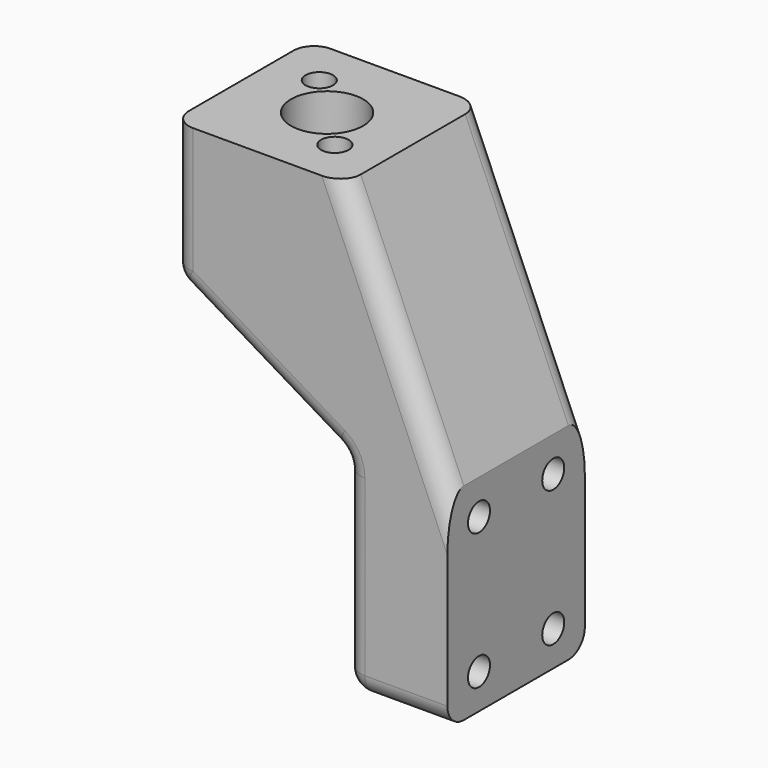
from build123d import *

# Parameters (mm, degrees)
F0_W      = 25
F0_H      = 20
F0_W_2    = 15
F0_H_2    = 30
F1_DEPTH  = 25
F2_R      = 5.25
F3_DEPTH  = 65.001
F4_R      = 2
F5_DEPTH  = 25
F6_R      = 3
F7_R      = 2
F8_DEPTH  = 65.001
F9_R      = 3.25
F10_DEPTH = 55.001


with BuildPart() as f1:
    # F0 (on Front) → F1 (new body)
    with BuildSketch(Plane.XZ):
        Polygon((12.5, 10), (12.5, -10), (-12.5, -10), (12.5, -25), (27.5, -25), align=None)
        Rectangle(F0_W, F0_H)
        with Locations((20, -40)):
            Rectangle(F0_W_2, F0_H_2)
    extrude(amount=F1_DEPTH)

    # F2 (on face) → F3 (cut, through all)
    with BuildSketch(Plane.XY.offset(10)):
        with Locations((0, -12.5)):
            Circle(F2_R)
    extrude(amount=-F3_DEPTH, mode=Mode.SUBTRACT)

    # F4 (on face) → F5 (cut)
    with BuildSketch(Plane(origin=(12.5, 0, 0), x_dir=(0, -1, 0), z_dir=(-1, 0, 0))):
        with Locations((19.25, -30.1)):
            Circle(F4_R)
        with Locations((5.75, -49.9)):
            Circle(F4_R)
        with Locations((5.75, -30.1)):
            Circle(F4_R)
        with Locations((19.25, -49.9)):
            Circle(F4_R)
    extrude(amount=-F5_DEPTH, mode=Mode.SUBTRACT)

    # F6
    f6_edges = [f1.edges().sort_by_distance(p)[0] for p in [
        (-12.5, -25, 0),
        (-12.5, 0, 0),
        (-12.5, -12.5, -10),
        (0, -25, -17.5),
        (0, 0, -17.5),
        (12.5, -12.5, -25),
        (12.5, -12.5, -55),
        (20, -25, -7.5),
        (20, 0, -7.5),
        (20, -25, -55),
        (20, 0, -55),
        (12.5, 0, -40),
        (12.5, -25, -40),
    ]]
    fillet(f6_edges, radius=F6_R)

    # F7 (on face) → F8 (cut, through all)
    with BuildSketch(Plane.XY.offset(10)):
        with Locations((-5.6568542495, -6.8431457505)):
            Circle(F7_R)
        with Locations((5.6568542495, -18.1568542495)):
            Circle(F7_R)
    extrude(amount=-F8_DEPTH, mode=Mode.SUBTRACT)

    # F9 (on Top) → F10 (cut, through all)
    with BuildSketch(Plane.XY):
        with Locations((-5.6611075997, -6.9247833453)):
            Circle(F9_R)
        with Locations((5.6935697794, -18.1814264506)):
            Circle(F9_R)
    extrude(amount=-F10_DEPTH, mode=Mode.SUBTRACT)


solid = f1.part
